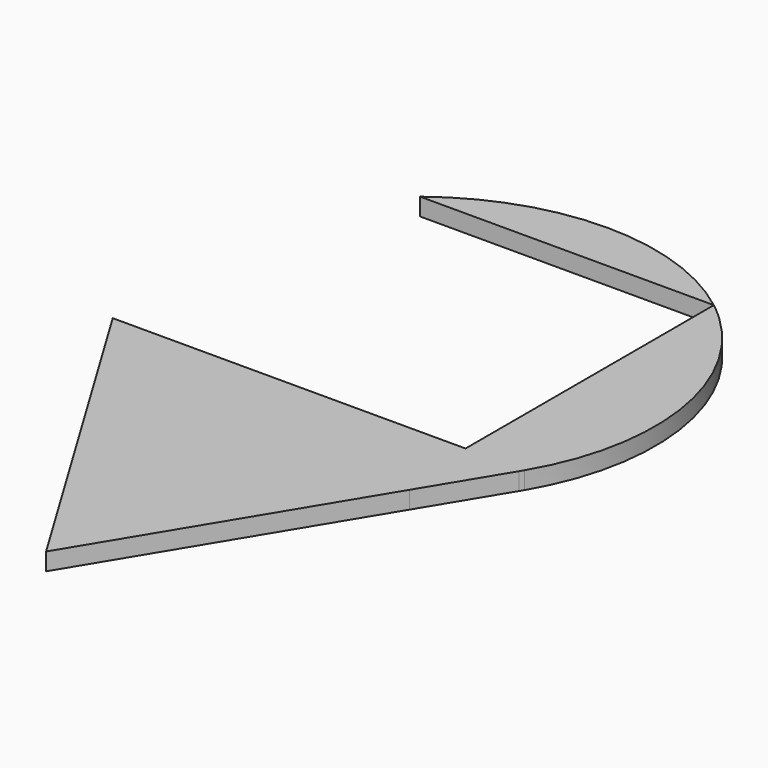
from build123d import *

# Parameters (mm, degrees)
F1_DEPTH = 3.175
F2_DEPTH = 6.35


# Not quite as in the source:
# - a feature names something its author has since deleted; it is built from what else it names


with BuildPart() as f1:
    # F0 (on Top) → F1 (new body)
    with BuildSketch(Plane.XY):
        with BuildLine():
            ThreePointArc((-0.0123727477, 68.6), (-26.7, 77.7594), (-53.3876272523, 68.6))
            Line((-53.3876272523, 68.6), (-0.0123727477, 68.6))
        make_face()
    extrude(amount=F1_DEPTH)


with BuildPart() as f1b:
    # F0 (on Top) → F1, piece 2 (new body)
    with BuildSketch(Plane.XY):
        Polygon((0, 12.1924446831), (-53.4, 12.1924446831), (-64.1162457533, 12.1924446831), (-63.6671424385, 11.4494020146), (-55.1402698288, -2.6583321515), (-26.7, -49.7128367424), (1.7402698288, -2.6583321515), (10.2671424385, 11.4494020146), (10.7162457533, 12.1924446831), (3.175, 12.1924446831), align=None)
        with BuildLine():
            Line((-53.4, 0), (-53.4, 0.0096303846))
            ThreePointArc((-53.4, 0.0096303846), (-53.3938140605, 0.0048146343), (-53.3876272523, 0))
            Line((-53.3876272523, 0), (-53.4, 0))
        make_face(mode=Mode.SUBTRACT)
        with BuildLine():
            ThreePointArc((-0.0123727477, 0), (-0.0061859395, 0.0048146343), (0, 0.0096303846))
            Line((0, 0.0096303846), (0, 0))
            Line((0, 0), (-0.0123727477, 0))
        make_face(mode=Mode.SUBTRACT)
        with BuildLine():
            ThreePointArc((3.175, 65.8626967061), (1.6203585098, 67.2647803305), (0, 68.5903696154))
            Line((0, 68.5903696154), (0, 12.1924446831))
            Line((0, 12.1924446831), (3.175, 12.1924446831))
            Line((3.175, 12.1924446831), (3.175, 65.8626967061))
        make_face()
        with BuildLine():
            ThreePointArc((10.7162457533, 12.1924446831), (16.3366347059, 40.3471085281), (3.175, 65.8626967061))
            Line((3.175, 65.8626967061), (3.175, 12.1924446831))
            Line((3.175, 12.1924446831), (10.7162457533, 12.1924446831))
        make_face()
    extrude(amount=F1_DEPTH)

    # F0 (on Top) → F2 (join)
    with BuildSketch(Plane.XY):
        with BuildLine():
            ThreePointArc((-53.3876272523, 0), (-53.3938140605, 0.0048146343), (-53.4, 0.0096303846))
            Line((-53.4, 0.0096303846), (-53.4, 0))
            Line((-53.4, 0), (-53.3876272523, 0))
        make_face()
    extrude(amount=F2_DEPTH)


solid = Compound([f1.part, f1b.part])
